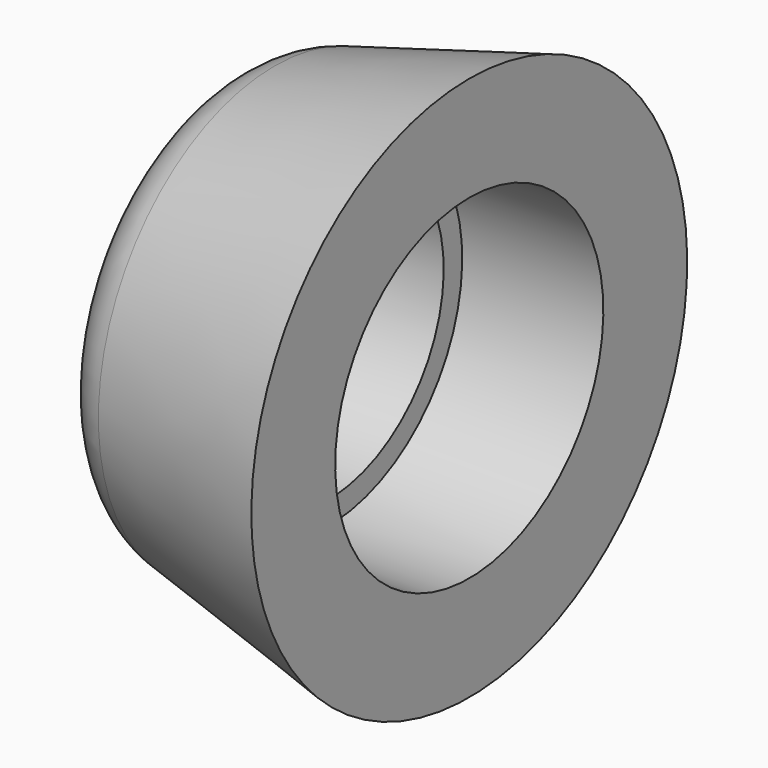
from build123d import *


# Not quite as in the source:
# - a feature names something its author has since deleted; it is built from what else it names


with BuildPart() as f1:
    # F0 (on Front) → F1 (revolve)
    with BuildSketch(Plane.XZ):
        with BuildLine():
            Line((0, 7.540625), (0, 12.2555))
            Line((0, 12.2555), (-8.7592504682, 9.9084659107))
            ThreePointArc((-8.7592504682, 9.9084659107), (-10.4563968554, 8.7744689494), (-11.1125, 6.8416514123))
            Line((-11.1125, 6.8416514123), (-11.1125, 6.49986))
            Line((-11.1125, 6.49986), (-6.35, 6.49986))
            Line((-6.35, 6.49986), (-6.35, 7.540625))
            Line((-6.35, 7.540625), (0, 7.540625))
        make_face()
    revolve(axis=Axis((5.2561350167, 0, 0), (1, 0, 0)))


solid = f1.part
